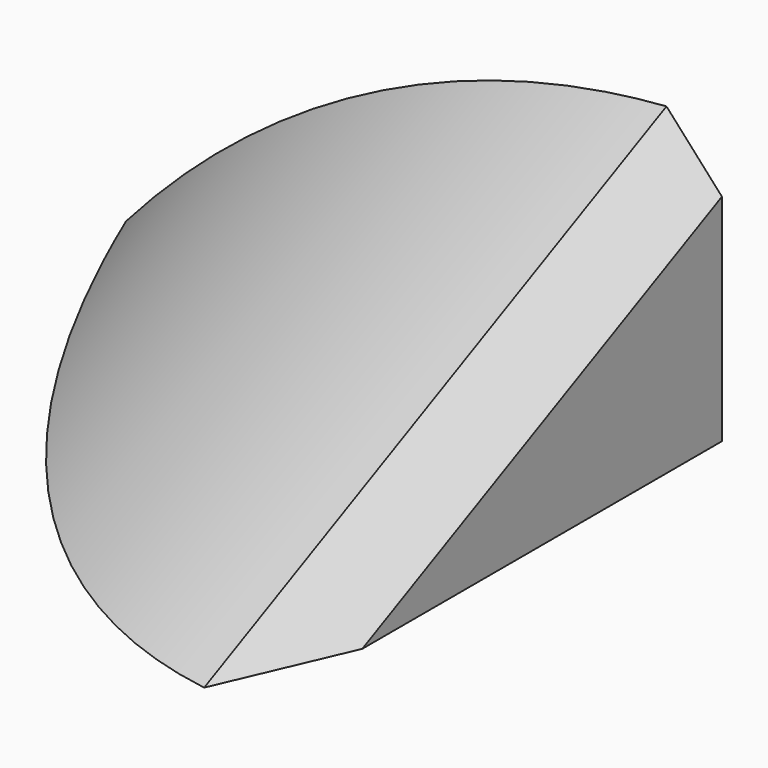
from build123d import *

# Parameters (mm, degrees)
F3_DEPTH    = 76.2
F4_SIZE     = 5.08
F5_T1_DEPTH = 438.8719745558


# Not quite as in the source:
# - a fillet or chamfer that OpenCascade refuses, or shapes differently, is made with other operations: its cross-section is extruded or revolved along the edge and cut away or added
# - a feature of the source that left no trace in its solid (it failed there, or was rolled back) is left out


with BuildPart() as f3:
    # F2 (on Right) → F3 (new body)
    with BuildSketch(Plane.YZ):
        Polygon((-52.9574006796, 0), (0, 0), (0, 25.36736615), align=None)
    extrude(amount=-F3_DEPTH)

    # F4
    f4_edges = [f3.edges().sort_by_distance(p)[0] for p in [
        (0, -26.4787, 12.683683),
    ]]
    chamfer(f4_edges, length=F4_SIZE)

    # F5: fillet of radius 76.2 on 1 edges, made by hand

    # F5_s2 → F5_t1 (cut)
    with BuildSketch(Plane(origin=(0, 181.3074352717, 86.8489018954), x_dir=(1, 0, 0), z_dir=(0, -0.9018694789, -0.4320086144))):
        with BuildLine():
            ThreePointArc((-5.08, 22.8780532919), (-55.6486118425, -1.0979149163), (-76.2, -53.1524248074))
            Line((-76.2, -53.1524248074), (-76.2, 22.8780532919))
            Line((-76.2, 22.8780532919), (-5.08, 22.8780532919))
        make_face()
    extrude(amount=F5_T1_DEPTH, mode=Mode.SUBTRACT)


solid = f3.part
